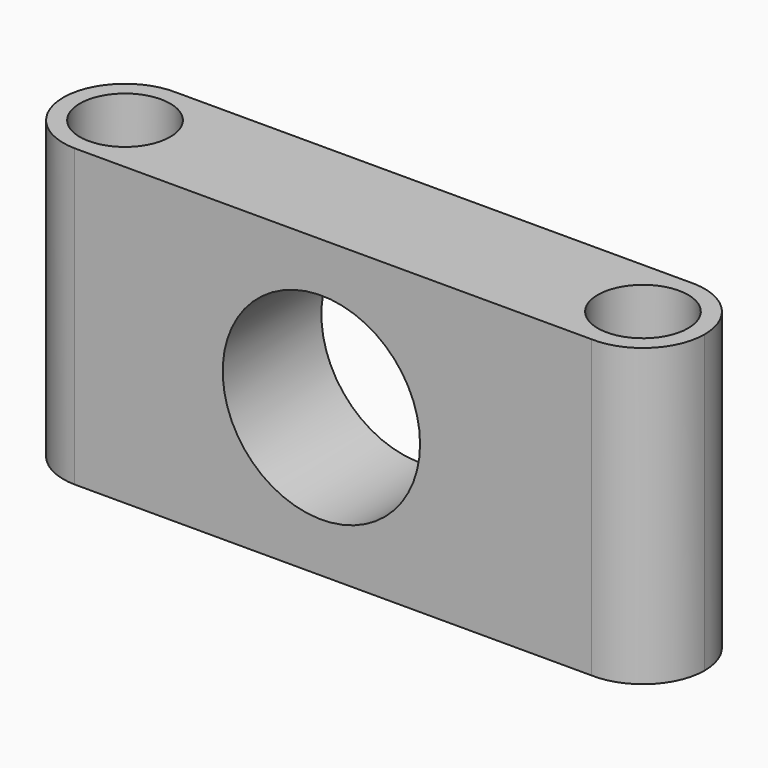
from build123d import *

# Parameters (mm, degrees)
F0_R     = 2.75
F1_DEPTH = 18
F2_R     = 6
F3_DEPTH = 7.5005674408


# Not quite as in the source:
# - a feature names something its author has since deleted; it is built from what else it names


with BuildPart() as f1:
    # F0 (on Top) → F1 (new body)
    with BuildSketch(Plane.XY):
        with BuildLine():
            ThreePointArc((-14.8575540239, 3.74907491), (-12.2599082251, 2.6220374098), (-11.1908445954, 0))
            Line((-11.1908445954, 0), (12.8071008226, 0))
            ThreePointArc((12.8071008226, 0), (13.8537114507, 2.599708945), (16.4096532115, 3.74907491))
            Line((16.4096532115, 3.74907491), (-14.8575540239, 3.74907491))
        make_face()
        with BuildLine():
            ThreePointArc((-14.8838884093, -3.7495674408), (-12.269133, -2.6314363285), (-11.1908445954, 0))
            ThreePointArc((-11.1908445954, 0), (-12.2599082251, 2.6220374098), (-14.8575540239, 3.74907491))
            ThreePointArc((-14.8575540239, 3.74907491), (-18.6901888916, 0.0701238113), (-14.9978007816, -3.7495674408))
            Line((-14.9978007816, -3.7495674408), (-14.8838884093, -3.7495674408))
        make_face()
        with Locations((-14.9408445954, 0)):
            Circle(F0_R, mode=Mode.SUBTRACT)
        with BuildLine():
            ThreePointArc((16.4096532115, 3.74907491), (13.8537114507, 2.599708945), (12.8071008226, 0))
            ThreePointArc((12.8071008226, 0), (13.858191018, -2.60436268), (16.4225626025, -3.7495674408))
            ThreePointArc((16.4225626025, -3.7495674408), (19.1635180845, -2.7009643866), (20.3112099866, 0))
            ThreePointArc((20.3112099866, 0), (19.2645993584, 2.599708945), (16.7086575976, 3.74907491))
            Line((16.7086575976, 3.74907491), (16.4096532115, 3.74907491))
        make_face()
        with Locations((16.5591554046, 0)):
            Circle(F0_R, mode=Mode.SUBTRACT)
        with BuildLine():
            Line((12.8071008226, 0), (-11.1908445954, 0))
            ThreePointArc((-11.1908445954, 0), (-12.269133, -2.6314363285), (-14.8838884093, -3.7495674408))
            Line((-14.8838884093, -3.7495674408), (16.4225626025, -3.7495674408))
            ThreePointArc((16.4225626025, -3.7495674408), (13.858191018, -2.60436268), (12.8071008226, 0))
        make_face()
    extrude(amount=F1_DEPTH)

    # F2 (on face) → F3 (cut, through all)
    with BuildSketch(Plane.XZ.offset(3.7495674408)):
        with Locations((0.0021992184, 9)):
            Circle(F2_R)
    extrude(amount=-F3_DEPTH, mode=Mode.SUBTRACT)


solid = f1.part
